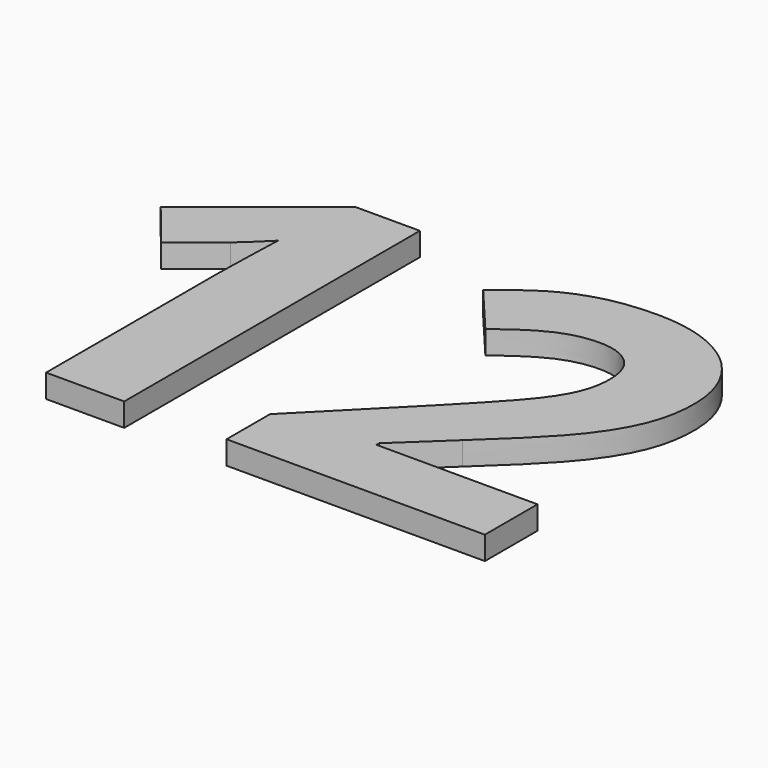
from build123d import *

# Parameters (mm, degrees)
F0_TEXT_SIZE = 111.1111111111
F1_DEPTH     = 5


# Not quite as in the source:
# - Text() gives the source's letters only with a copy of the font that has no kerning and outlines rounded to 1/6400 em; it was checked with that copy


with BuildPart() as f1:
    # F0 (on Top) → F1 (new body)
    with BuildSketch(Plane.XY):
        with Locations((-71.1594222461, -50.4347826087)):
            Text('12', F0_TEXT_SIZE, font='Open Sans', font_style=FontStyle.BOLD, text_align=(TextAlign.LEFT, TextAlign.BOTTOM))
    extrude(amount=F1_DEPTH)


solid = f1.part
